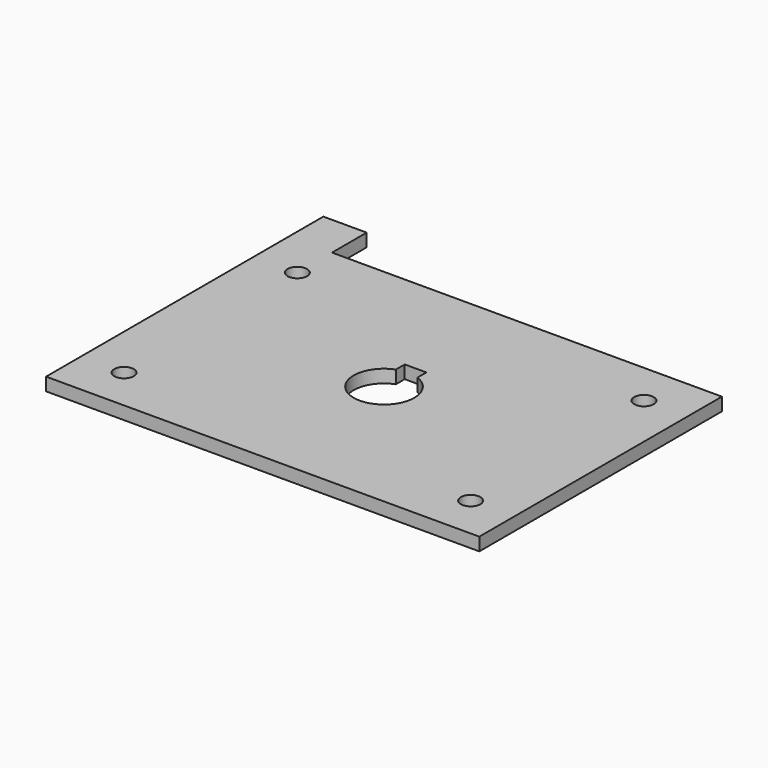
from build123d import *

# Parameters (mm, degrees)
F0_R     = 2.25
F0_W     = 10
F0_H     = 10
F1_DEPTH = 3


# Not quite as in the source:
# - a feature names something its author has since deleted; it is built from what else it names


with BuildPart() as f1:
    # F0 (on Top) → F1 (new body)
    with BuildSketch(Plane.XY):
        Polygon((-50, -39.9732751399), (50, -39.9732751399), (50, 30.0267248601), (-40, 30.0267248601), (-50, 30.0267248601), align=None)
        with Locations((-40, -29.9732751399)):
            Circle(F0_R, mode=Mode.SUBTRACT)
        with Locations((40, -29.9732751399)):
            Circle(F0_R, mode=Mode.SUBTRACT)
        with BuildLine():
            Line((2.5, 4.1267248601), (2.5, 1.5650732754))
            ThreePointArc((2.5, 1.5650732754), (5.7662812973, -1.0046481733), (7, -4.9732751399))
            ThreePointArc((7, -4.9732751399), (-3.9686269666, -10.7395564373), (-2.5, 1.5650732754))
            Line((-2.5, 1.5650732754), (-2.5, 4.1267248601))
            Line((-2.5, 4.1267248601), (2.5, 4.1267248601))
        make_face(mode=Mode.SUBTRACT)
        with Locations((-40, 20.0267248601)):
            Circle(F0_R, mode=Mode.SUBTRACT)
        with Locations((40, 20.0267248601)):
            Circle(F0_R, mode=Mode.SUBTRACT)
        with Locations((-45, 35.0267248601)):
            Rectangle(F0_W, F0_H)
    extrude(amount=F1_DEPTH)


solid = f1.part
